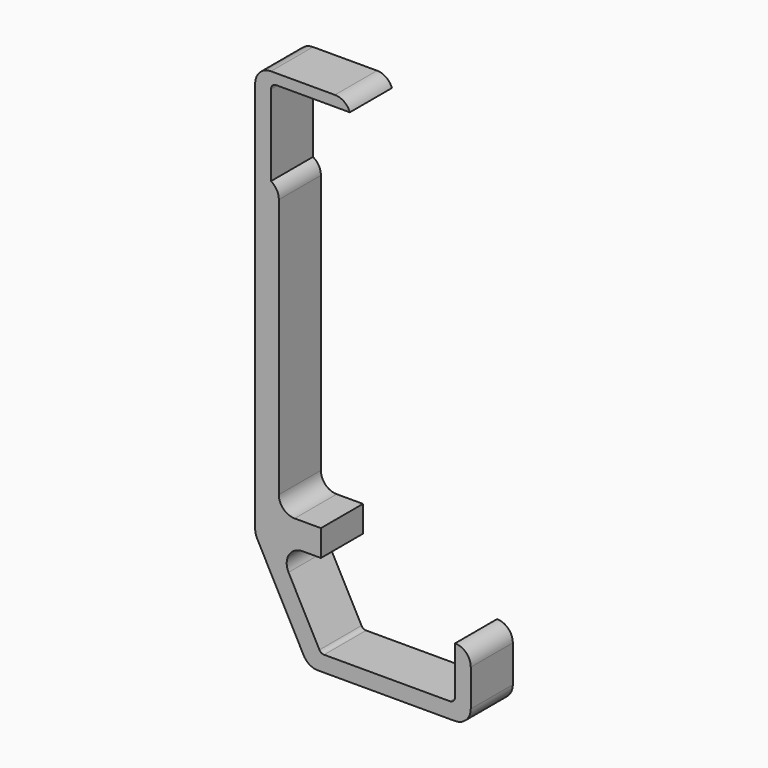
from build123d import *

# Parameters (mm, degrees)
F1_DEPTH    = 10
F2_T1_DEPTH = 25
F2_T3_DEPTH = 24.1421356237
F2_T5_DEPTH = 19.0165664987
F2_T7_DEPTH = 13.7370663506
F3_R        = 1
F4_T1_DEPTH = 10
F4_T3_DEPTH = 10
F4_T5_DEPTH = 22.9903810568


# Not quite as in the source:
# - a fillet or chamfer that OpenCascade refuses, or shapes differently, is made with other operations: its cross-section is extruded or revolved along the edge and cut away or added
# - a feature names something its author has since deleted; it is built from what else it names


with BuildPart() as f1:
    # F0 (on Front) → F1 (new body)
    with BuildSketch(Plane.XZ):
        Polygon((-50, 8.2), (-35, 8.2), (-35, 10.2), (-53, 10.2), (-53, -68.2), (-49, -68.2), (-49, -63.2), (-48.5, -63.2), (-48.5, -8.2), (-50, -8.2), align=None)
        Polygon((-49, -68.2), (-53, -68.2), (-44.5, -84.2), (-40.5, -84.2), align=None)
        Polygon((-12, -74.2), (-15, -74.2), (-15, -84.2), (-40.5, -84.2), (-44.5, -84.2), (-42.90625, -87.2), (-12, -87.2), align=None)
        Polygon((-40.5, -68.2), (-40.5, -63.2), (-48.5, -63.2), (-49, -63.2), (-49, -68.2), align=None)
    extrude(amount=F1_DEPTH)

    # F2: fillet of radius 3 on 6 edges, made by hand

    # F2_s2 → F2_t1 (cut)
    with BuildSketch(Plane.XZ.offset(-7.5)):
        with BuildLine():
            ThreePointArc((-50, 10.2), (-52.1213203436, 9.3213203436), (-53, 7.2))
            Line((-53, 7.2), (-53, 10.2))
            Line((-53, 10.2), (-50, 10.2))
        make_face()
        with BuildLine():
            ThreePointArc((-12, -77.2), (-12.8786796564, -75.0786796564), (-15, -74.2))
            Line((-15, -74.2), (-12, -74.2))
            Line((-12, -74.2), (-12, -77.2))
        make_face()
        with BuildLine():
            ThreePointArc((-15, -87.2), (-12.8786796564, -86.3213203436), (-12, -84.2))
            Line((-12, -84.2), (-12, -87.2))
            Line((-12, -87.2), (-15, -87.2))
        make_face()
    extrude(amount=F2_T1_DEPTH, mode=Mode.SUBTRACT)

    # F2_s4 → F2_t3 (cut)
    with BuildSketch(Plane.XZ.offset(-7.0710678119)):
        with BuildLine():
            ThreePointArc((-35, 8.2), (-36.0963763172, 9.6494897428), (-37.8284271247, 10.2))
            Line((-37.8284271247, 10.2), (-35, 10.2))
            Line((-35, 10.2), (-35, 8.2))
        make_face()
    extrude(amount=F2_T3_DEPTH, mode=Mode.SUBTRACT)

    # F2_s6 → F2_t5 (cut)
    with BuildSketch(Plane.XZ.offset(-4.5082832494)):
        with BuildLine():
            ThreePointArc((-43.7522838586, -85.6074656779), (-42.648511507, -86.7712251004), (-41.1029367003, -87.2))
            Line((-41.1029367003, -87.2), (-42.90625, -87.2))
            Line((-42.90625, -87.2), (-43.7522838586, -85.6074656779))
        make_face()
    extrude(amount=F2_T5_DEPTH, mode=Mode.SUBTRACT)

    # F2_s8 → F2_t7 (cut)
    with BuildSketch(Plane.XZ.offset(-1.8685331753)):
        with BuildLine():
            ThreePointArc((-53, -67.4525867299), (-52.9110171311, -68.1778310077), (-52.6493471584, -68.8600524078))
            Line((-52.6493471584, -68.8600524078), (-53, -68.2))
            Line((-53, -68.2), (-53, -67.4525867299))
        make_face()
    extrude(amount=F2_T7_DEPTH, mode=Mode.SUBTRACT)

    # F3
    f3_edges = [f1.edges().sort_by_distance(p)[0] for p in [
        (-40.5, -5, -84.2),
        (-15, -5, -84.2),
        (-50, -5, 8.2),
    ]]
    fillet(f3_edges, radius=F3_R)

    # F4: fillet of radius 3 on 3 edges, made by hand

    # F4_s2 → F4_t1 (join)
    with BuildSketch(Plane.XZ):
        with BuildLine():
            ThreePointArc((-46.6585338586, -72.6074656779), (-46.5804118006, -69.6544251933), (-44.0091867003, -68.2))
            Line((-44.0091867003, -68.2), (-49, -68.2))
            Line((-49, -68.2), (-46.6585338586, -72.6074656779))
        make_face()
    extrude(amount=F4_T1_DEPTH)

    # F4_s4 → F4_t3 (join)
    with BuildSketch(Plane.XZ):
        with BuildLine():
            ThreePointArc((-45.5, -63.2), (-47.6213203436, -62.3213203436), (-48.5, -60.2))
            Line((-48.5, -60.2), (-48.5, -63.2))
            Line((-48.5, -63.2), (-45.5, -63.2))
        make_face()
    extrude(amount=F4_T3_DEPTH)

    # F4_s6 → F4_t5 (cut)
    with BuildSketch(Plane.XZ.offset(-6.4951905284)):
        with BuildLine():
            ThreePointArc((-50, -8.2), (-48.9019237886, -9.2980762114), (-48.5, -10.7980762114))
            Line((-48.5, -10.7980762114), (-48.5, -8.2))
            Line((-48.5, -8.2), (-50, -8.2))
        make_face()
    extrude(amount=F4_T5_DEPTH, mode=Mode.SUBTRACT)


solid = f1.part
